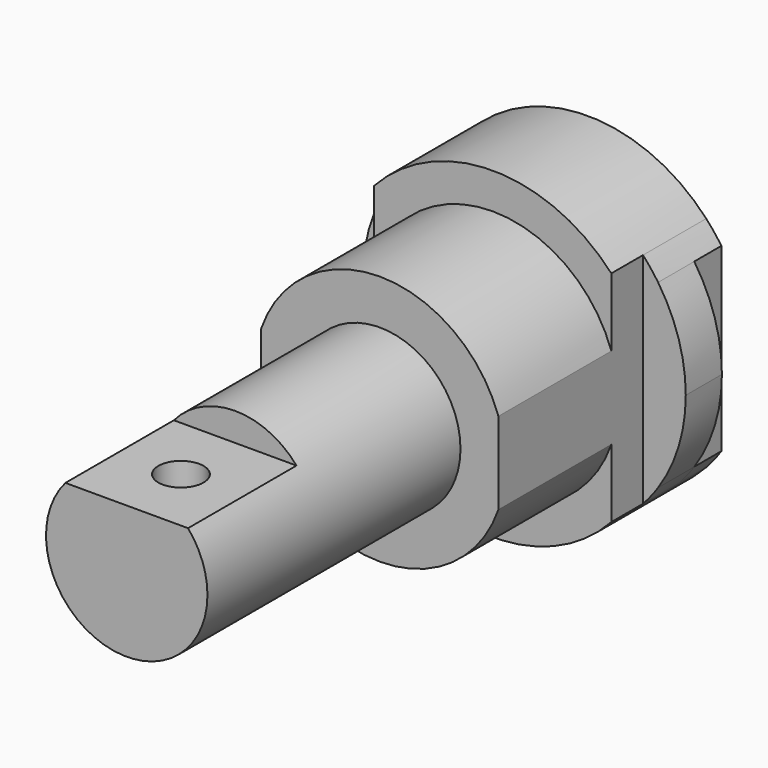
from build123d import *
from build123d import SkipClean  # not in build123d's __all__

# Parameters (mm, degrees)
F1_DEPTH = 6
F2_DEPTH = 8
F3_DEPTH = 15
F4_DEPTH = 72
F5_DEPTH = 96
F6_DEPTH = 40
F7_R     = 4
F8_DEPTH = 25


# Not quite as in the source:
# - after a boolean that leaves OpenCascade's solid faulty, fix() repairs it


with BuildPart() as f1:
    # F0 (on Front) → F1 (new body)
    with BuildSketch(Plane.XZ):
        with BuildLine():
            Line((-21, 7.2767180102), (-21, 19.3786125664))
            ThreePointArc((-21, 19.3786125664), (-22.4015502975, 17.7398187497), (-23.6755279772, 16))
            Line((-23.6755279772, 16), (-23.6755279772, -16))
            ThreePointArc((-23.6755279772, -16), (-22.4015502975, -17.7398187497), (-21, -19.3786125664))
            Line((-21, -19.3786125664), (-21, -7.2767180102))
            ThreePointArc((-21, -7.2767180102), (-22.225, 0), (-21, 7.2767180102))
        make_face()
        with BuildLine():
            Line((-21, -7.2767180102), (-21, 7.2767180102))
            ThreePointArc((-21, 7.2767180102), (-22.225, 0), (-21, -7.2767180102))
        make_face()
        with BuildLine():
            Line((21, 7.2767180102), (21, 19.3786125664))
            ThreePointArc((21, 19.3786125664), (0, 28.575), (-21, 19.3786125664))
            Line((-21, 19.3786125664), (-21, 7.2767180102))
            ThreePointArc((-21, 7.2767180102), (0, 22.225), (21, 7.2767180102))
        make_face()
        with BuildLine():
            Line((21, -7.2767180102), (21, 7.2767180102))
            ThreePointArc((21, 7.2767180102), (0, 22.225), (-21, 7.2767180102))
            Line((-21, 7.2767180102), (-21, -7.2767180102))
            ThreePointArc((-21, -7.2767180102), (0, -22.225), (21, -7.2767180102))
        make_face()
        with BuildLine():
            ThreePointArc((10.8581766425, 9.29), (13.4046157017, 4.9518055181), (14.29, 0))
            ThreePointArc((14.29, 0), (-4.9518055181, -13.4046157017), (-10.8581766425, 9.29))
            ThreePointArc((-10.8581766425, 9.29), (0, 14.29), (10.8581766425, 9.29))
        make_face(mode=Mode.SUBTRACT)
        with BuildLine():
            ThreePointArc((-21, -19.3786125664), (0, -28.575), (21, -19.3786125664))
            Line((21, -19.3786125664), (21, -7.2767180102))
            ThreePointArc((21, -7.2767180102), (0, -22.225), (-21, -7.2767180102))
            Line((-21, -7.2767180102), (-21, -19.3786125664))
        make_face()
        with BuildLine():
            ThreePointArc((22.225, 0), (21.9166104245, 3.6895545124), (21, 7.2767180102))
            Line((21, 7.2767180102), (21, -7.2767180102))
            ThreePointArc((21, -7.2767180102), (21.9166104245, -3.6895545124), (22.225, 0))
        make_face()
        with BuildLine():
            Line((23.6755279772, -16), (23.6755279772, 16))
            ThreePointArc((23.6755279772, 16), (22.4015502975, 17.7398187497), (21, 19.3786125664))
            Line((21, 19.3786125664), (21, 7.2767180102))
            ThreePointArc((21, 7.2767180102), (21.9166104245, 3.6895545124), (22.225, 0))
            ThreePointArc((22.225, 0), (21.9166104245, -3.6895545124), (21, -7.2767180102))
            Line((21, -7.2767180102), (21, -19.3786125664))
            ThreePointArc((21, -19.3786125664), (22.4015502975, -17.7398187497), (23.6755279772, -16))
        make_face()
        with BuildLine():
            ThreePointArc((-10.8581766425, 9.29), (-4.9518055181, -13.4046157017), (14.29, 0))
            ThreePointArc((14.29, 0), (13.4046157017, 4.9518055181), (10.8581766425, 9.29))
            Line((10.8581766425, 9.29), (-10.8581766425, 9.29))
        make_face()
        with BuildLine():
            Line((-10.8581766425, 9.29), (10.8581766425, 9.29))
            ThreePointArc((10.8581766425, 9.29), (0, 14.29), (-10.8581766425, 9.29))
        make_face()
    extrude(amount=-F1_DEPTH)

    # F0 (on Front) → F2 (join)
    with BuildSketch(Plane.XZ):
        with BuildLine():
            Line((21, -7.2767180102), (21, 7.2767180102))
            ThreePointArc((21, 7.2767180102), (0, 22.225), (-21, 7.2767180102))
            Line((-21, 7.2767180102), (-21, -7.2767180102))
            ThreePointArc((-21, -7.2767180102), (0, -22.225), (21, -7.2767180102))
        make_face()
        with BuildLine():
            ThreePointArc((10.8581766425, 9.29), (13.4046157017, 4.9518055181), (14.29, 0))
            ThreePointArc((14.29, 0), (-4.9518055181, -13.4046157017), (-10.8581766425, 9.29))
            ThreePointArc((-10.8581766425, 9.29), (0, 14.29), (10.8581766425, 9.29))
        make_face(mode=Mode.SUBTRACT)
        with BuildLine():
            ThreePointArc((-10.8581766425, 9.29), (-4.9518055181, -13.4046157017), (14.29, 0))
            ThreePointArc((14.29, 0), (13.4046157017, 4.9518055181), (10.8581766425, 9.29))
            Line((10.8581766425, 9.29), (-10.8581766425, 9.29))
        make_face()
        with BuildLine():
            Line((21, 7.2767180102), (21, 19.3786125664))
            ThreePointArc((21, 19.3786125664), (0, 28.575), (-21, 19.3786125664))
            Line((-21, 19.3786125664), (-21, 7.2767180102))
            ThreePointArc((-21, 7.2767180102), (0, 22.225), (21, 7.2767180102))
        make_face()
        with BuildLine():
            ThreePointArc((-21, -19.3786125664), (0, -28.575), (21, -19.3786125664))
            Line((21, -19.3786125664), (21, -7.2767180102))
            ThreePointArc((21, -7.2767180102), (0, -22.225), (-21, -7.2767180102))
            Line((-21, -7.2767180102), (-21, -19.3786125664))
        make_face()
        with BuildLine():
            ThreePointArc((23.6755279772, -16), (27.3226905424, -8.3666723687), (28.575, 0))
            ThreePointArc((28.575, 0), (27.3226905424, 8.3666723687), (23.6755279772, 16))
            Line((23.6755279772, 16), (23.6755279772, -16))
        make_face()
        with BuildLine():
            Line((-23.6755279772, -16), (-23.6755279772, 16))
            ThreePointArc((-23.6755279772, 16), (-28.575, 0), (-23.6755279772, -16))
        make_face()
        with BuildLine():
            Line((23.6755279772, -16), (23.6755279772, 16))
            ThreePointArc((23.6755279772, 16), (22.4015502975, 17.7398187497), (21, 19.3786125664))
            Line((21, 19.3786125664), (21, 7.2767180102))
            ThreePointArc((21, 7.2767180102), (21.9166104245, 3.6895545124), (22.225, 0))
            ThreePointArc((22.225, 0), (21.9166104245, -3.6895545124), (21, -7.2767180102))
            Line((21, -7.2767180102), (21, -19.3786125664))
            ThreePointArc((21, -19.3786125664), (22.4015502975, -17.7398187497), (23.6755279772, -16))
        make_face()
        with BuildLine():
            Line((-21, 7.2767180102), (-21, 19.3786125664))
            ThreePointArc((-21, 19.3786125664), (-22.4015502975, 17.7398187497), (-23.6755279772, 16))
            Line((-23.6755279772, 16), (-23.6755279772, -16))
            ThreePointArc((-23.6755279772, -16), (-22.4015502975, -17.7398187497), (-21, -19.3786125664))
            Line((-21, -19.3786125664), (-21, -7.2767180102))
            ThreePointArc((-21, -7.2767180102), (-22.225, 0), (-21, 7.2767180102))
        make_face()
        with BuildLine():
            Line((-10.8581766425, 9.29), (10.8581766425, 9.29))
            ThreePointArc((10.8581766425, 9.29), (0, 14.29), (-10.8581766425, 9.29))
        make_face()
        with BuildLine():
            Line((-21, -7.2767180102), (-21, 7.2767180102))
            ThreePointArc((-21, 7.2767180102), (-22.225, 0), (-21, -7.2767180102))
        make_face()
        with BuildLine():
            ThreePointArc((22.225, 0), (21.9166104245, 3.6895545124), (21, 7.2767180102))
            Line((21, 7.2767180102), (21, -7.2767180102))
            ThreePointArc((21, -7.2767180102), (21.9166104245, -3.6895545124), (22.225, 0))
        make_face()
    with SkipClean():  # cleaning this boolean's faces spoils the solid; the shape is the same uncleaned
        extrude(amount=F2_DEPTH)

    # F0 (on Front) → F3 (join)
    with BuildSketch(Plane.XZ):
        with BuildLine():
            Line((21, -7.2767180102), (21, 7.2767180102))
            ThreePointArc((21, 7.2767180102), (0, 22.225), (-21, 7.2767180102))
            Line((-21, 7.2767180102), (-21, -7.2767180102))
            ThreePointArc((-21, -7.2767180102), (0, -22.225), (21, -7.2767180102))
        make_face()
        with BuildLine():
            ThreePointArc((10.8581766425, 9.29), (13.4046157017, 4.9518055181), (14.29, 0))
            ThreePointArc((14.29, 0), (-4.9518055181, -13.4046157017), (-10.8581766425, 9.29))
            ThreePointArc((-10.8581766425, 9.29), (0, 14.29), (10.8581766425, 9.29))
        make_face(mode=Mode.SUBTRACT)
        with BuildLine():
            ThreePointArc((-10.8581766425, 9.29), (-4.9518055181, -13.4046157017), (14.29, 0))
            ThreePointArc((14.29, 0), (13.4046157017, 4.9518055181), (10.8581766425, 9.29))
            Line((10.8581766425, 9.29), (-10.8581766425, 9.29))
        make_face()
        with BuildLine():
            Line((21, 7.2767180102), (21, 19.3786125664))
            ThreePointArc((21, 19.3786125664), (0, 28.575), (-21, 19.3786125664))
            Line((-21, 19.3786125664), (-21, 7.2767180102))
            ThreePointArc((-21, 7.2767180102), (0, 22.225), (21, 7.2767180102))
        make_face()
        with BuildLine():
            ThreePointArc((-21, -19.3786125664), (0, -28.575), (21, -19.3786125664))
            Line((21, -19.3786125664), (21, -7.2767180102))
            ThreePointArc((21, -7.2767180102), (0, -22.225), (-21, -7.2767180102))
            Line((-21, -7.2767180102), (-21, -19.3786125664))
        make_face()
        with BuildLine():
            Line((-10.8581766425, 9.29), (10.8581766425, 9.29))
            ThreePointArc((10.8581766425, 9.29), (0, 14.29), (-10.8581766425, 9.29))
        make_face()
    extrude(amount=F3_DEPTH)

    add(f1.part.fix(), mode=Mode.REPLACE)

    # F0 (on Front) → F4 (join)
    with BuildSketch(Plane.XZ):
        with BuildLine():
            ThreePointArc((-10.8581766425, 9.29), (-4.9518055181, -13.4046157017), (14.29, 0))
            ThreePointArc((14.29, 0), (13.4046157017, 4.9518055181), (10.8581766425, 9.29))
            Line((10.8581766425, 9.29), (-10.8581766425, 9.29))
        make_face()
        with BuildLine():
            Line((-10.8581766425, 9.29), (10.8581766425, 9.29))
            ThreePointArc((10.8581766425, 9.29), (0, 14.29), (-10.8581766425, 9.29))
        make_face()
    extrude(amount=F4_DEPTH)

    # F0 (on Front) → F5 (join)
    with BuildSketch(Plane.XZ):
        with BuildLine():
            ThreePointArc((-10.8581766425, 9.29), (-4.9518055181, -13.4046157017), (14.29, 0))
            ThreePointArc((14.29, 0), (13.4046157017, 4.9518055181), (10.8581766425, 9.29))
            Line((10.8581766425, 9.29), (-10.8581766425, 9.29))
        make_face()
    extrude(amount=F5_DEPTH)

    # F0 (on Front) → F6 (join)
    with BuildSketch(Plane.XZ):
        with BuildLine():
            Line((21, -7.2767180102), (21, 7.2767180102))
            ThreePointArc((21, 7.2767180102), (0, 22.225), (-21, 7.2767180102))
            Line((-21, 7.2767180102), (-21, -7.2767180102))
            ThreePointArc((-21, -7.2767180102), (0, -22.225), (21, -7.2767180102))
        make_face()
        with BuildLine():
            ThreePointArc((10.8581766425, 9.29), (13.4046157017, 4.9518055181), (14.29, 0))
            ThreePointArc((14.29, 0), (-4.9518055181, -13.4046157017), (-10.8581766425, 9.29))
            ThreePointArc((-10.8581766425, 9.29), (0, 14.29), (10.8581766425, 9.29))
        make_face(mode=Mode.SUBTRACT)
        with BuildLine():
            ThreePointArc((-10.8581766425, 9.29), (-4.9518055181, -13.4046157017), (14.29, 0))
            ThreePointArc((14.29, 0), (13.4046157017, 4.9518055181), (10.8581766425, 9.29))
            Line((10.8581766425, 9.29), (-10.8581766425, 9.29))
        make_face()
        with BuildLine():
            Line((-10.8581766425, 9.29), (10.8581766425, 9.29))
            ThreePointArc((10.8581766425, 9.29), (0, 14.29), (-10.8581766425, 9.29))
        make_face()
    extrude(amount=F6_DEPTH)

    # F7 (on face) → F8 (cut)
    with BuildSketch(Plane.XY.offset(9.29)):
        with Locations((0, -84)):
            Circle(F7_R)
    extrude(amount=-F8_DEPTH, mode=Mode.SUBTRACT)


solid = f1.part
